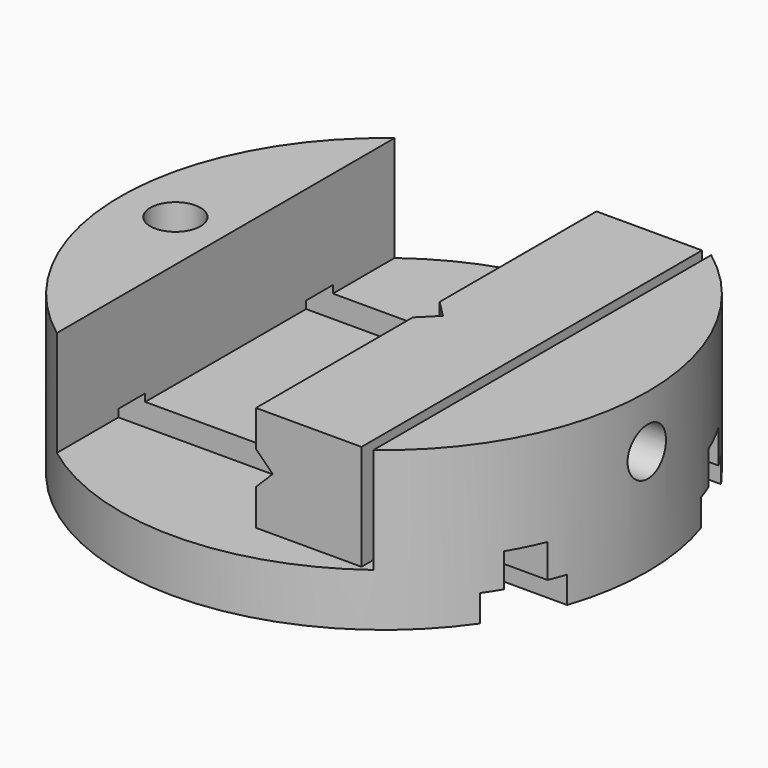
from build123d import *

# Parameters (mm, degrees)
F0_R          = 50
F1_DEPTH      = 30
F2_W          = 60
F2_H          = 104.775
F3_DEPTH      = 20
F4_W          = 12.7
F4_H          = 5.08
F5_DEPTH      = 50.001
F5_DEPTH_BACK = 50.001
F6_W          = 6.35
F6_H          = 12.7
F7_DEPTH      = 50.001
F7_DEPTH_BACK = 50.001
F8_R          = 4.55
F9_DEPTH      = 50.001
F10_R         = 2.15
F11_DEPTH     = 4.826
F12_R         = 2.15
F13_DEPTH     = 5.174
F15_W         = 20
F15_H         = 20
F16_DEPTH     = 40.3225
F17_R         = 3.81
F18_DEPTH     = 12
F20_DEPTH     = 90.3235001
F22_DEPTH     = 30.0010001
F23_R         = 4.7625
F24_DEPTH     = 30.0010001


with BuildPart() as f1:
    # F0 (on Top) → F1 (new body)
    with BuildSketch(Plane.XY):
        Circle(F0_R)
    extrude(amount=F1_DEPTH)

    # F2 (on face) → F3 (cut)
    with BuildSketch(Plane.XY.offset(30)):
        Rectangle(F2_W, F2_H)
    extrude(amount=-F3_DEPTH, mode=Mode.SUBTRACT)

    # F4 (on Right) → F5 (cut, two sides)
    with BuildSketch(Plane.YZ) as f5_sk:
        with Locations((-22.225, 2.54)):
            Rectangle(F4_W, F4_H)
        with Locations((22.225, 2.54)):
            Rectangle(F4_W, F4_H)
    extrude(amount=-F5_DEPTH, mode=Mode.SUBTRACT)
    extrude(f5_sk.sketch, amount=F5_DEPTH_BACK, mode=Mode.SUBTRACT)

    # F6 (on Right) → F7 (cut, two sides)
    with BuildSketch(Plane.YZ) as f7_sk:
        with Locations((-22.225, 5.08)):
            Rectangle(F6_W, F6_H)
        with Locations((22.225, 5.08)):
            Rectangle(F6_W, F6_H)
    extrude(amount=-F7_DEPTH, mode=Mode.SUBTRACT)
    extrude(f7_sk.sketch, amount=F7_DEPTH_BACK, mode=Mode.SUBTRACT)

    # F8 (on Right) → F9 (cut, through all)
    with BuildSketch(Plane.YZ):
        with Locations((0, 20)):
            Circle(F8_R)
    extrude(amount=F9_DEPTH, mode=Mode.SUBTRACT)

    # F23 (on face) → F24 (cut, through all)
    with BuildSketch(Plane.XY.offset(30)):
        with Locations((-39.525, 0)):
            Circle(F23_R)
    extrude(amount=-F24_DEPTH, mode=Mode.SUBTRACT)


with BuildPart() as f11:
    # F10 (on face) → F11 (new body)
    with BuildSketch(Plane(origin=(0, 0, 0), x_dir=(1, 0, 0), z_dir=(0, 0, -1))):
        with BuildLine():
            Line((6.8875, -28.4988), (29.1125, -28.4988))
            ThreePointArc((29.1125, -28.4988), (30.2350320151, -28.0338320151), (30.7, -26.9113))
            Line((30.7, -26.9113), (30.7, -17.5387))
            ThreePointArc((30.7, -17.5387), (30.2350320151, -16.4161679849), (29.1125, -15.9512))
            Line((29.1125, -15.9512), (6.8875, -15.9512))
            ThreePointArc((6.8875, -15.9512), (5.7649679849, -16.4161679849), (5.3, -17.5387))
            Line((5.3, -17.5387), (5.3, -26.9113))
            ThreePointArc((5.3, -26.9113), (5.7649679849, -28.0338320151), (6.8875, -28.4988))
        make_face()
        with Locations((18, -22.225)):
            Circle(F10_R, mode=Mode.SUBTRACT)
    extrude(amount=-F11_DEPTH)

    # F12 (on face) → F13 (join, through all)
    with BuildSketch(Plane.XY.offset(4.826)):
        with BuildLine():
            ThreePointArc((8, 20.6883), (8.4649679849, 19.5657679849), (9.5875, 19.1008))
            Line((9.5875, 19.1008), (26.4125, 19.1008))
            ThreePointArc((26.4125, 19.1008), (27.5350320151, 19.5657679849), (28, 20.6883))
            Line((28, 20.6883), (28, 23.7617))
            ThreePointArc((28, 23.7617), (27.5350320151, 24.8842320151), (26.4125, 25.3492))
            Line((26.4125, 25.3492), (9.5875, 25.3492))
            ThreePointArc((9.5875, 25.3492), (8.4649679849, 24.8842320151), (8, 23.7617))
            Line((8, 23.7617), (8, 20.6883))
        make_face()
        with Locations((18, 22.225)):
            Circle(F12_R, mode=Mode.SUBTRACT)
    extrude(amount=F13_DEPTH)


with BuildPart() as f14_1:
    # F14: instance of F11
    add(f11.part.mirror(Plane.XZ))


with BuildPart() as f16:
    # F15 (on Front) → F16 (new body, symmetric)
    with BuildSketch(Plane.XZ):
        with Locations((18, 20)):
            Rectangle(F15_W, F15_H)
    extrude(amount=F16_DEPTH, both=True)

    # F17 (on face) → F18 (cut)
    with BuildSketch(Plane.YZ.offset(28)):
        with Locations((0, 20)):
            Circle(F17_R)
    extrude(amount=-F18_DEPTH, mode=Mode.SUBTRACT)

    # F19 (on face) → F20 (cut, through all)
    with BuildSketch(Plane.XZ.offset(40.3225)):
        Polygon((8, 23.175), (8, 16.825), (11.175, 20), align=None)
    extrude(amount=-F20_DEPTH, mode=Mode.SUBTRACT)

    # F21 (on face) → F22 (cut, through all)
    with BuildSketch(Plane.XY.offset(30)):
        Polygon((11.175, 0), (8, 3.175), (8, -3.175), align=None)
    extrude(amount=-F22_DEPTH, mode=Mode.SUBTRACT)


solid = Compound([f1.part, f11.part, f14_1.part, f16.part])
